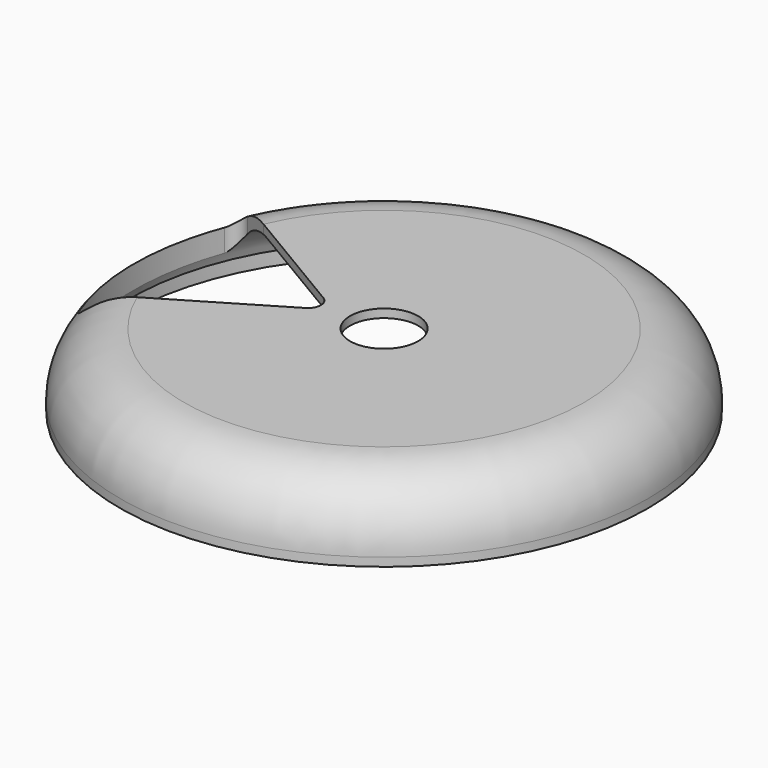
from build123d import *

# Parameters (mm, degrees)
F0_R      = 62
F1_DEPTH  = 17
F2_R      = 60
F3_DEPTH  = 15
F4_R      = 14.99999
F5_R      = 61
F6_DEPTH  = 4
F8_DEPTH  = 25
F9_R      = 3
F10_R     = 8
F11_DEPTH = 25


# Not quite as in the source:
# - a fillet or chamfer is up to 0.001 mm smaller than in the source, because OpenCascade refuses the exact size


with BuildPart() as f1:
    # F0 (on Top) → F1 (new body)
    with BuildSketch(Plane.XY):
        Circle(F0_R)
    extrude(amount=F1_DEPTH)

    # F2 (on face) → F3 (cut)
    with BuildSketch(Plane(origin=(0, 0, 0), x_dir=(1, 0, 0), z_dir=(0, 0, -1))):
        Circle(F2_R)
    extrude(amount=-F3_DEPTH, mode=Mode.SUBTRACT)

    # F4 (radius 15 in the source; OpenCascade refuses exactly that, so slightly less here)
    f4_edges = [f1.edges().sort_by_distance(p)[0] for p in [
        (-60, 0, 15),
        (-62, 0, 17),
    ]]
    fillet(f4_edges, radius=F4_R)

    # F5 (on face) → F6 (cut)
    with BuildSketch(Plane(origin=(0, 0, 0), x_dir=(1, 0, 0), z_dir=(0, 0, -1))):
        Circle(F5_R)
    extrude(amount=-F6_DEPTH, mode=Mode.SUBTRACT)

    # F7 (on face) → F8 (cut)
    with BuildSketch(Plane.XY.offset(17)):
        with BuildLine():
            Line((-43.1747773956, -18.5725479362), (-12, 0))
            Line((-12, 0), (-43.1747773956, 18.5725479362))
            ThreePointArc((-43.1747773956, 18.5725479362), (-47.00001, 0), (-43.1747773956, -18.5725479362))
        make_face()
        with BuildLine():
            ThreePointArc((-43.1747773956, -18.5725479362), (-47.00001, 0), (-43.1747773956, 18.5725479362))
            Line((-43.1747773956, 18.5725479362), (-53.2366762866, 24.5669804581))
            ThreePointArc((-53.2366762866, 24.5669804581), (-58.8026071187, 0), (-53.2366762866, -24.5669804581))
            Line((-53.2366762866, -24.5669804581), (-43.1747773956, -18.5725479362))
        make_face()
    extrude(amount=-F8_DEPTH, mode=Mode.SUBTRACT)

    # F9
    f9_edges = [f1.edges().sort_by_distance(p)[0] for p in [
        (-12, 0, 16),
        (-53.236676, -24.56698, 8.865114),
        (-53.236676, 24.56698, 8.865114),
    ]]
    fillet(f9_edges, radius=F9_R)

    # F10 (on face) → F11 (cut)
    with BuildSketch(Plane.XY.offset(17)):
        Circle(F10_R)
    extrude(amount=-F11_DEPTH, mode=Mode.SUBTRACT)


solid = f1.part
